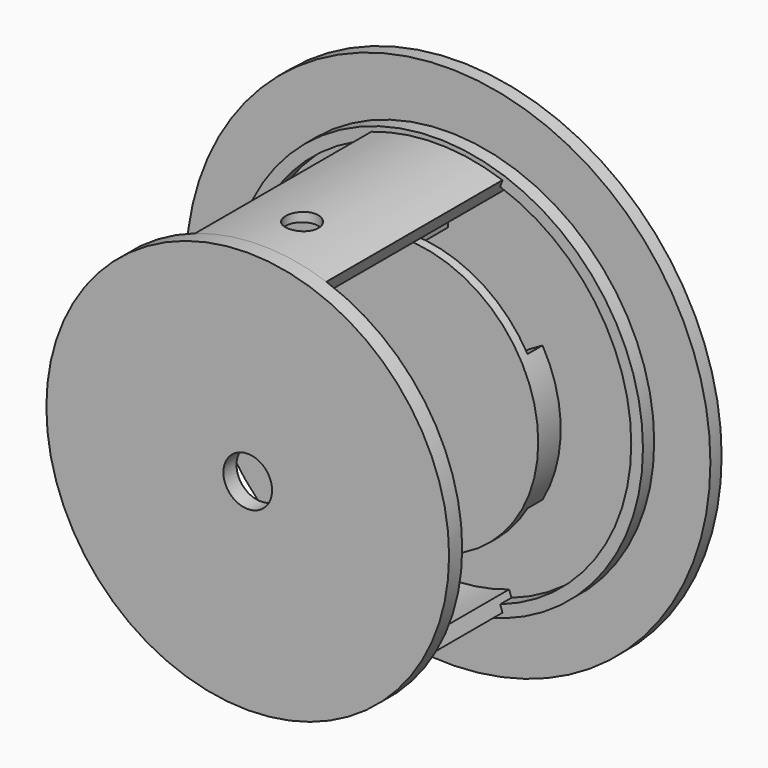
from build123d import *

# Parameters (mm, degrees)
F0_R           = 28
F1_DEPTH       = 1.5
F3_DEPTH       = 5.1
F5_DEPTH       = 25
F6_R           = 21.5
F7_DEPTH       = 1.75
F8_R           = 2.6
F9_DEPTH       = 25
F10_R          = 1.975
F11_DEPTH      = 30
F13_END_RADIUS = 21.5
F12_R          = 3.75
F12_R_2        = 1.875
F13_REACH      = 38.6076017178
F14_W          = 15
F14_H          = 26.820743024
F15_DEPTH      = 25
F15_DEPTH_BACK = 25
F16_R          = 14.5
F17_DEPTH      = 1
F19_DEPTH      = 2
F21_R          = 22.5
F21_R_2        = 20.5
F22_DEPTH      = 1
F23_R          = 22
F23_R_2        = 20.75
F24_DEPTH      = 1.5
F25_R          = 3.1
F26_DEPTH      = 5.5
F27_R          = 1.75
F28_REACH      = 12.4507474683
F29_R          = 30
F29_R_2        = 29
F30_DEPTH      = 25


with BuildPart() as f1:
    # F0 (on Front) → F1 (new body)
    with BuildSketch(Plane.XZ):
        Circle(F0_R)
    extrude(amount=F1_DEPTH)

    # F2 (on face) → F3 (join)
    with BuildSketch(Plane.XZ.offset(1.5)):
        with BuildLine():
            ThreePointArc((0, -13), (-13, 0), (0, 13))
            Line((0, 13), (0, 14.5))
            ThreePointArc((0, 14.5), (-14.5, 0), (0, -14.5))
            Line((0, -14.5), (0, -13))
        make_face()
    extrude(amount=F3_DEPTH)

    # F4 (on face) → F5 (join)
    with BuildSketch(Plane.XZ.offset(1.5)):
        with BuildLine():
            Line((6.5113630891, 18.910371512), (6.9997153208, 20.3286493754))
            ThreePointArc((6.9997153208, 20.3286493754), (0, 21.5), (-6.9997153208, 20.3286493754))
            Line((-6.9997153208, 20.3286493754), (-6.5113630891, 18.910371512))
            ThreePointArc((-6.5113630891, 18.910371512), (0, 20), (6.5113630891, 18.910371512))
        make_face()
        with BuildLine():
            ThreePointArc((6.5113630891, -18.910371512), (0, -20), (-6.5113630891, -18.910371512))
            Line((-6.5113630891, -18.910371512), (-6.9997153208, -20.3286493754))
            ThreePointArc((-6.9997153208, -20.3286493754), (0, -21.5), (6.9997153208, -20.3286493754))
            Line((6.9997153208, -20.3286493754), (6.5113630891, -18.910371512))
        make_face()
    extrude(amount=F5_DEPTH)

    # F6 (on face) → F7 (join)
    with BuildSketch(Plane.XZ.offset(26.5)):
        Circle(F6_R)
    extrude(amount=F7_DEPTH)

    # F8 (on face) → F9 (cut)
    with BuildSketch(Plane.XZ.offset(28.25)):
        Circle(F8_R)
    extrude(amount=-F9_DEPTH, mode=Mode.SUBTRACT)

    # F10 (on Top) → F11 (cut)
    with BuildSketch(Plane.XY):
        with Locations((0, -20.5)):
            Circle(F10_R)
    extrude(amount=-F11_DEPTH, mode=Mode.SUBTRACT)

    f13_end = (Plane.ZX.offset(-14) * Cylinder(F13_END_RADIUS, 245.3825308212, mode=Mode.PRIVATE)).faces().sort_by_distance((0, -14, -21.5))[0]
    # F12 (on Top) → F13 (join, up to the whole of a round face its end follows)
    with BuildSketch(Plane.XY):
        with Locations((0, -20.5)):
            Circle(F12_R)
        with Locations((0, -20.5)):
            Circle(F12_R_2, mode=Mode.SUBTRACT)
    f13_long = extrude(amount=-F13_REACH, mode=Mode.PRIVATE)
    add(split(f13_long, bisect_by=f13_end, keep=Keep.BOTTOM, mode=Mode.PRIVATE))

    # F14 (on Right) → F15 (cut, two sides)
    with BuildSketch(Plane.YZ) as f15_sk:
        with Locations((-17.75, 0)):
            Rectangle(F14_W, F14_H)
    extrude(amount=-F15_DEPTH, mode=Mode.SUBTRACT)
    extrude(f15_sk.sketch, amount=F15_DEPTH_BACK, mode=Mode.SUBTRACT)

    # F16 (on face) → F17 (join)
    with BuildSketch(Plane.XZ.offset(6.6)):
        Circle(F16_R)
    extrude(amount=F17_DEPTH)

    # F18 (on face) → F19 (join)
    with BuildSketch(Plane(origin=(0, -6.6, 0), x_dir=(-1, 0, 0), z_dir=(0, 1, 0))):
        with BuildLine():
            Line((-11.0418238983, 6.375), (-12.5573683549, 7.25))
            ThreePointArc((-12.5573683549, 7.25), (-14.5, 0), (-12.5573683549, -7.25))
            Line((-12.5573683549, -7.25), (-11.0418238983, -6.375))
            ThreePointArc((-11.0418238983, -6.375), (-12.75, 0), (-11.0418238983, 6.375))
        make_face()
    extrude(amount=F19_DEPTH)

    # F21 (on face) → F22 (join)
    with BuildSketch(Plane(origin=(0, 0, 0), x_dir=(-1, 0, 0), z_dir=(0, 1, 0))):
        Circle(F21_R)
        Circle(F21_R_2, mode=Mode.SUBTRACT)
    extrude(amount=F22_DEPTH)

    # F23 (on face) → F24 (join)
    with BuildSketch(Plane.XZ.offset(1.5)):
        Circle(F23_R)
        Circle(F23_R_2, mode=Mode.SUBTRACT)
    extrude(amount=F24_DEPTH)

    # F25 (on offset) → F26 (cut)
    with BuildSketch(Plane.XY.offset(15)):
        with Locations((0, -21)):
            Circle(F25_R)
    extrude(amount=F26_DEPTH, mode=Mode.SUBTRACT)

    f28_end = f1.faces().sort_by_distance((17.5034836447, -27.1584498842, 12.4851135478))[0]
    # F27 (on face) → F28 (cut, up to a face of the model that its end follows)
    with BuildSketch(Plane(origin=(0, 0, 20.5), x_dir=(1, 0, 0), z_dir=(0, 0, -1))):
        with Locations((0, 21)):
            Circle(F27_R)
    f28_long = extrude(amount=-F28_REACH, mode=Mode.PRIVATE)
    add(split(f28_long, bisect_by=f28_end, keep=Keep.BOTTOM, mode=Mode.PRIVATE), mode=Mode.SUBTRACT)

    # F29 (on face) → F30 (cut)
    with BuildSketch(Plane.XZ.offset(1.5)):
        Circle(F29_R)
        Circle(F29_R_2, mode=Mode.SUBTRACT)
    extrude(amount=F30_DEPTH, mode=Mode.SUBTRACT)


solid = f1.part
